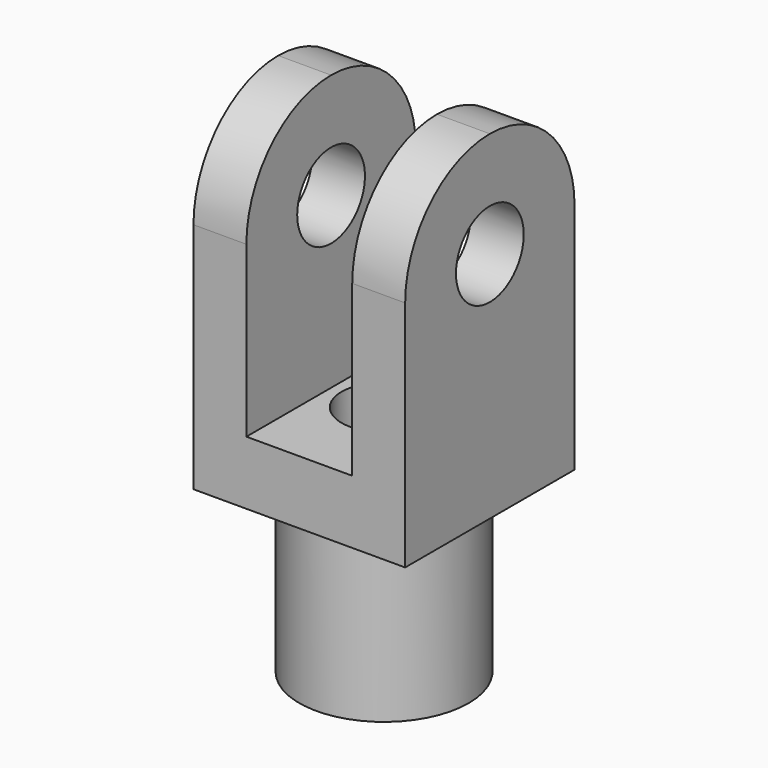
from build123d import *

# Parameters (mm, degrees)
F1_DEPTH = 25
F2_R     = 20
F2_R_2   = 10
F3_DEPTH = 40
F4_DEPTH = 15
F5_R     = 10
F6_DEPTH = 56.6
F7_R     = 24.99999


# Not quite as in the source:
# - a fillet or chamfer is up to 0.001 mm smaller than in the source, because OpenCascade refuses the exact size


with BuildPart() as f1:
    # F0 (on Front) → F1 (new body, symmetric)
    with BuildSketch(Plane.XZ):
        Polygon((-12.5, 40), (-25, 40), (-25, -40), (25, -40), (25, 40), (12.5, 40), (12.5, -25), (-12.5, -25), align=None)
    extrude(amount=F1_DEPTH, both=True)

    # F2 (on face) → F3 (join)
    with BuildSketch(Plane(origin=(0, 0, -40), x_dir=(1, 0, 0), z_dir=(0, 0, -1))):
        Circle(F2_R)
        Circle(F2_R_2, mode=Mode.SUBTRACT)
    extrude(amount=F3_DEPTH)

    # F2 (on face) → F4 (cut)
    with BuildSketch(Plane(origin=(0, 0, -40), x_dir=(1, 0, 0), z_dir=(0, 0, -1))):
        Circle(F2_R_2)
    extrude(amount=-F4_DEPTH, mode=Mode.SUBTRACT)

    # F5 (on face) → F6 (cut)
    with BuildSketch(Plane(origin=(-25, 0, 0), x_dir=(0, -1, 0), z_dir=(-1, 0, 0))):
        with Locations((0, 15)):
            Circle(F5_R)
    extrude(amount=-F6_DEPTH, mode=Mode.SUBTRACT)

    # F7 (radius 25 in the source; OpenCascade refuses exactly that, so slightly less here)
    f7_edges = [f1.edges().sort_by_distance(p)[0] for p in [
        (18.75, 25, 40),
        (18.75, -25, 40),
        (-18.75, 25, 40),
        (-18.75, -25, 40),
    ]]
    fillet(f7_edges, radius=F7_R)


solid = f1.part
